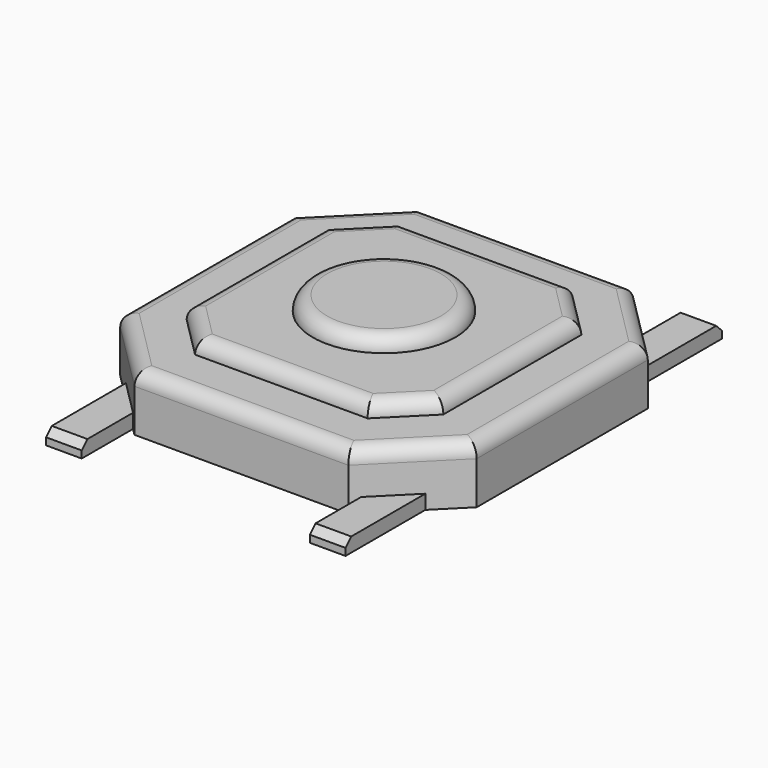
from build123d import *

# Parameters (mm, degrees)
F1_DEPTH   = 0.8
F0_W       = 0.5
F0_H       = 0.8
F2_DEPTH   = 0.2
F3_R       = 0.2
F5_DEPTH   = 0.2
F6_R       = 0.19999
F7_R       = 1
F8_DEPTH   = 0.2
F9_R       = 0.19999
F10_SIZE   = 0.1
F10_2_SIZE = 0.1
F10_3_SIZE = 0.1
F10_4_SIZE = 0.1


# Not quite as in the source:
# - a fillet or chamfer is up to 0.001 mm smaller than in the source, because OpenCascade refuses the exact size


with BuildPart() as f1:
    # F0 (on Top) → F1 (new body)
    with BuildSketch(Plane.XY):
        Polygon((-2.1, 1.9), (-2.5, 1.5), (-2.5, -1.5), (-2.1, -1.9), (-1.6, -2.4), (-1.5, -2.5), (1.5, -2.5), (1.6, -2.4), (2.1, -1.9), (2.5, -1.5), (2.5, 1.5), (2.1, 1.9), (1.6, 2.4), (1.5, 2.5), (-1.5, 2.5), (-1.6, 2.4), align=None)
    extrude(amount=F1_DEPTH)

    # F3
    f3_edges = [f1.edges().sort_by_distance(p)[0] for p in [
        (-2, 2, 0.8),
        (-2.5, 0, 0.8),
        (-2, -2, 0.8),
        (0, -2.5, 0.8),
        (2, -2, 0.8),
        (2.5, 0, 0.8),
        (2, 2, 0.8),
        (0, 2.5, 0.8),
    ]]
    fillet(f3_edges, radius=F3_R)

    # F4 (on face) → F5 (join)
    with BuildSketch(Plane.XY.offset(0.8)):
        Polygon((1.2100505063, 1.8), (-1.2100505063, 1.8), (-1.8, 1.2100505063), (-1.8, -1.2100505063), (-1.2100505063, -1.8), (1.2100505063, -1.8), (1.8, -1.2100505063), (1.8, 1.2100505063), align=None)
    extrude(amount=F5_DEPTH)

    # F6 (radius 0.2 in the source; OpenCascade refuses exactly that, so slightly less here)
    f6_edges = [f1.edges().sort_by_distance(p)[0] for p in [
        (1.505025, 1.505025, 1),
        (0, 1.8, 1),
        (-1.505025, 1.505025, 1),
        (-1.8, 0, 1),
        (-1.505025, -1.505025, 1),
        (0, -1.8, 1),
        (1.505025, -1.505025, 1),
        (1.8, 0, 1),
    ]]
    fillet(f6_edges, radius=F6_R)


with BuildPart() as f2:
    # F0 (on Top) → F2 (new body)
    with BuildSketch(Plane.XY):
        Polygon((-1.6, -2.4), (-2.1, -1.9), (-2.1, -2.5), (-1.6, -2.5), align=None)
        with Locations((-1.85, -2.9)):
            Rectangle(F0_W, F0_H)
    extrude(amount=F2_DEPTH)

    # F10#4
    f10_4_edges = [f2.edges().sort_by_distance(p)[0] for p in [
        (-1.85, -3.3, 0.2),
    ]]
    chamfer(f10_4_edges, length=F10_4_SIZE)


with BuildPart() as f2b:
    # F0 (on Top) → F2, piece 2 (new body)
    with BuildSketch(Plane.XY):
        with Locations((-1.85, 2.9)):
            Rectangle(F0_W, F0_H)
        Polygon((-1.6, 2.5), (-2.1, 2.5), (-2.1, 1.9), (-1.6, 2.4), align=None)
    extrude(amount=F2_DEPTH)

    # F10
    f10_edges = [f2b.edges().sort_by_distance(p)[0] for p in [
        (-1.85, 3.3, 0.2),
    ]]
    chamfer(f10_edges, length=F10_SIZE)


with BuildPart() as f2c:
    # F0 (on Top) → F2, piece 3 (new body)
    with BuildSketch(Plane.XY):
        with Locations((1.85, 2.9)):
            Rectangle(F0_W, F0_H)
        Polygon((2.1, 2.5), (1.6, 2.5), (1.6, 2.4), (2.1, 1.9), align=None)
    extrude(amount=F2_DEPTH)

    # F10#2
    f10_2_edges = [f2c.edges().sort_by_distance(p)[0] for p in [
        (1.85, 3.3, 0.2),
    ]]
    chamfer(f10_2_edges, length=F10_2_SIZE)


with BuildPart() as f2d:
    # F0 (on Top) → F2, piece 4 (new body)
    with BuildSketch(Plane.XY):
        Polygon((1.6, -2.4), (1.6, -2.5), (2.1, -2.5), (2.1, -1.9), align=None)
        with Locations((1.85, -2.9)):
            Rectangle(F0_W, F0_H)
    extrude(amount=F2_DEPTH)

    # F10#3
    f10_3_edges = [f2d.edges().sort_by_distance(p)[0] for p in [
        (1.85, -3.3, 0.2),
    ]]
    chamfer(f10_3_edges, length=F10_3_SIZE)


with BuildPart() as f8:
    # F7 (on face) → F8 (new body)
    with BuildSketch(Plane.XY.offset(1)):
        Circle(F7_R)
    extrude(amount=F8_DEPTH)

    # F9 (radius 0.2 in the source; OpenCascade refuses exactly that, so slightly less here)
    f9_edges = [f8.edges().sort_by_distance(p)[0] for p in [
        (-1, 0, 1.2),
    ]]
    fillet(f9_edges, radius=F9_R)


solid = Compound([f1.part, f2.part, f2b.part, f2c.part, f2d.part, f8.part])
